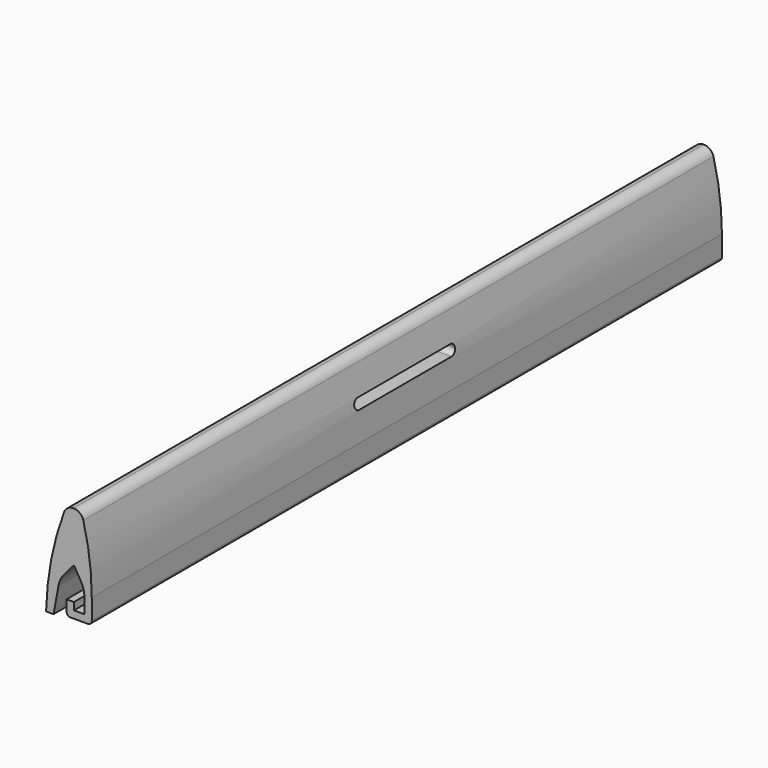
from build123d import *

# Parameters (mm, degrees)
F1_DEPTH = 75
F3_DEPTH = 12.5
F4_R     = 1.9


# Not quite as in the source:
# - ends of sketch curves that miss each other by under 0.0002 mm in the source are joined


with BuildPart() as f1:
    # F0 (on Front) → F1 (new body, symmetric)
    with BuildSketch(Plane.XZ):
        with BuildLine():
            Line((1.4, 9), (-1.4, 9))
            ThreePointArc((-1.4, 9), (-4.202341, -0.325046), (-5.3, -10))
            Line((-5.3, -10), (-3.876062, -10))
            Line((-3.876062, -10), (-2.921314, -4.859053))
            ThreePointArc((-2.921314, -4.859053), (-2.543024, -3.702321), (-1.874627, -2.685278))
            Line((-1.874627, -2.685278), (0, -0.522247))
            Line((0, -0.522247), (1.297343, -2.703488))
            ThreePointArc((1.297343, -2.703488), (1.821137, -3.934047), (2, -5.259431))
            Line((2, -5.259431), (2, -8.1))
            Line((2, -8.1), (0, -8.1))
            Line((0, -8.1), (0, -6.7))
            Line((0, -6.7), (-1.4, -6.7))
            Line((-1.4, -6.7), (-1.4, -8.75))
            ThreePointArc((-1.4, -8.75), (-1.18033, -9.28033), (-0.65, -9.5))
            Line((-0.65, -9.5), (2.65, -9.5))
            ThreePointArc((2.65, -9.5), (3.18033, -9.28033), (3.4, -8.75))
            Line((3.4, -8.75), (3.4, -4.874555))
            ThreePointArc((3.4, -4.874555), (2.897429, 2.134426), (1.4, 9))
        make_face()
    extrude(amount=F1_DEPTH, both=True)

    # F2 (on Right) → F3 (cut, symmetric)
    with BuildSketch(Plane.YZ):
        with BuildLine():
            ThreePointArc((12, 1.5), (11.707107, 2.207107), (11, 2.5))
            Line((11, 2.5), (-11, 2.5))
            ThreePointArc((-11, 2.5), (-11.707107, 2.207107), (-12, 1.5))
            ThreePointArc((-12, 1.5), (-11.707107, 0.792893), (-11, 0.5))
            Line((-11, 0.5), (11, 0.5))
            ThreePointArc((11, 0.5), (11.707107, 0.792893), (12, 1.5))
        make_face()
    extrude(amount=F3_DEPTH, both=True, mode=Mode.SUBTRACT)

    # F4
    f4_edges = [f1.edges().sort_by_distance(p)[0] for p in [
        (-1.4, 0, 9),
        (1.4, 0, 9),
    ]]
    fillet(f4_edges, radius=F4_R)


solid = f1.part
